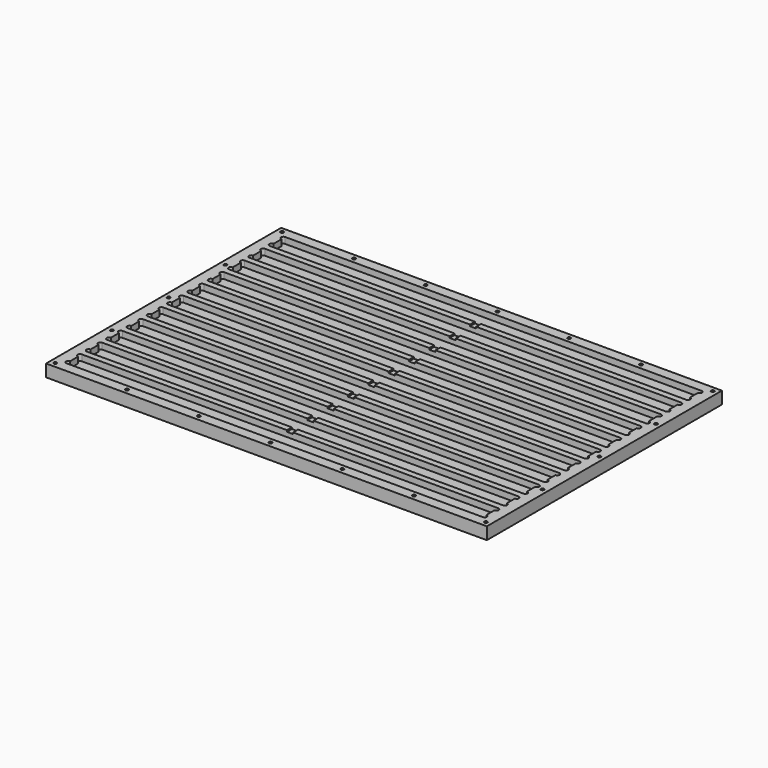
from build123d import *

# Parameters (mm, degrees)
F2_W      = 457.2
F2_H      = 304.8
F3_DEPTH  = 12.7
F4_W      = 431.8
F4_H      = 20.0152
F5_DEPTH  = 6.35
F7_D      = 3.3
F8_R      = 2.3876
F9_DEPTH  = 6.35
F10_W     = 6.35
F10_H     = 283.6672
F11_DEPTH = 1.5875


# Not quite as in the source:
# - a variable given as a bare number and used for a length is read in inches; the dataset says mm whatever the document's units were


with BuildPart() as f3:
    # F2 (on Top) → F3 (new body)
    with BuildSketch(Plane.XY):
        Rectangle(F2_W, F2_H)
    extrude(amount=F3_DEPTH)

    # F4 (on face) → F5 (cut)
    with BuildSketch(Plane.XY.offset(12.7)):
        with Locations((0, 131.826)):
            Rectangle(F4_W, F4_H)
        with Locations((0, 105.4608)):
            Rectangle(F4_W, F4_H)
        with Locations((0, 79.0956)):
            Rectangle(F4_W, F4_H)
        with Locations((0, 52.7304)):
            Rectangle(F4_W, F4_H)
        with Locations((0, 26.3652)):
            Rectangle(F4_W, F4_H)
        Rectangle(F4_W, F4_H)
        with Locations((0, -26.3652)):
            Rectangle(F4_W, F4_H)
        with Locations((0, -52.7304)):
            Rectangle(F4_W, F4_H)
        with Locations((0, -79.0956)):
            Rectangle(F4_W, F4_H)
        with Locations((0, -105.4608)):
            Rectangle(F4_W, F4_H)
        with Locations((0, -131.826)):
            Rectangle(F4_W, F4_H)
    extrude(amount=-F5_DEPTH, mode=Mode.SUBTRACT)

    # F7 (through all)
    with Locations(Plane.XY.offset(12.7)):
        with Locations((-223.3168, 147.1168), (-223.3168, 73.5584), (-223.3168, 0), (-223.3168, -73.5584), (-223.3168, -147.1168), (-148.8778666667, -147.1168), (-74.4389333333, -147.1168), (0, -147.1168), (74.4389333333, -147.1168), (148.8778666667, -147.1168), (223.3168, -147.1168), (223.3168, -73.5584), (223.3168, 0), (223.3168, 73.5584), (223.3168, 147.1168), (148.8778666667, 147.1168), (74.4389333333, 147.1168), (0, 147.1168), (-74.4389333333, 147.1168), (-148.8778666667, 147.1168)):
            Hole(F7_D / 2)

    # F8 (on face) → F9 (cut)
    with BuildSketch(Plane.XY.offset(12.7)):
        with Locations((-215.9, 33.9852)):
            Circle(F8_R)
        with Locations((-215.9, 45.1104)):
            Circle(F8_R)
        with Locations((-215.9, 60.3504)):
            Circle(F8_R)
        with Locations((-215.9, 86.7156)):
            Circle(F8_R)
        with Locations((-215.9, 71.4756)):
            Circle(F8_R)
        with Locations((-215.9, 97.8408)):
            Circle(F8_R)
        with Locations((-215.9, 113.0808)):
            Circle(F8_R)
        with Locations((-215.9, 124.206)):
            Circle(F8_R)
        with Locations((-215.9, 139.446)):
            Circle(F8_R)
        with Locations((-215.9, 18.7452)):
            Circle(F8_R)
        with Locations((-215.9, 7.62)):
            Circle(F8_R)
        with Locations((215.9, 7.62)):
            Circle(F8_R)
        with Locations((215.9, 18.7452)):
            Circle(F8_R)
        with Locations((215.9, 33.9852)):
            Circle(F8_R)
        with Locations((215.9, 45.1104)):
            Circle(F8_R)
        with Locations((215.9, 60.3504)):
            Circle(F8_R)
        with Locations((215.9, 71.4756)):
            Circle(F8_R)
        with Locations((215.9, 86.7156)):
            Circle(F8_R)
        with Locations((215.9, 97.8408)):
            Circle(F8_R)
        with Locations((215.9, 113.0808)):
            Circle(F8_R)
        with Locations((215.9, 124.206)):
            Circle(F8_R)
        with Locations((215.9, 139.446)):
            Circle(F8_R)
        with Locations((215.9, -7.62)):
            Circle(F8_R)
        with Locations((215.9, -18.7452)):
            Circle(F8_R)
        with Locations((215.9, -33.9852)):
            Circle(F8_R)
        with Locations((215.9, -45.1104)):
            Circle(F8_R)
        with Locations((215.9, -60.3504)):
            Circle(F8_R)
        with Locations((215.9, -71.4756)):
            Circle(F8_R)
        with Locations((215.9, -86.7156)):
            Circle(F8_R)
        with Locations((215.9, -97.8408)):
            Circle(F8_R)
        with Locations((215.9, -113.0808)):
            Circle(F8_R)
        with Locations((215.9, -124.206)):
            Circle(F8_R)
        with Locations((215.9, -139.446)):
            Circle(F8_R)
        with Locations((-215.9, -7.62)):
            Circle(F8_R)
        with Locations((-215.9, -18.7452)):
            Circle(F8_R)
        with Locations((-215.9, -33.9852)):
            Circle(F8_R)
        with Locations((-215.9, -45.1104)):
            Circle(F8_R)
        with Locations((-215.9, -60.3504)):
            Circle(F8_R)
        with Locations((-215.9, -71.4756)):
            Circle(F8_R)
        with Locations((-215.9, -97.8408)):
            Circle(F8_R)
        with Locations((-215.9, -86.7156)):
            Circle(F8_R)
        with Locations((-215.9, -139.446)):
            Circle(F8_R)
        with Locations((-215.9, -124.206)):
            Circle(F8_R)
        with Locations((-215.9, -113.0808)):
            Circle(F8_R)
    extrude(amount=-F9_DEPTH, mode=Mode.SUBTRACT)

    # F10 (on face) → F11 (cut)
    with BuildSketch(Plane.XY.offset(12.7)):
        Rectangle(F10_W, F10_H)
    extrude(amount=-F11_DEPTH, mode=Mode.SUBTRACT)


solid = f3.part
